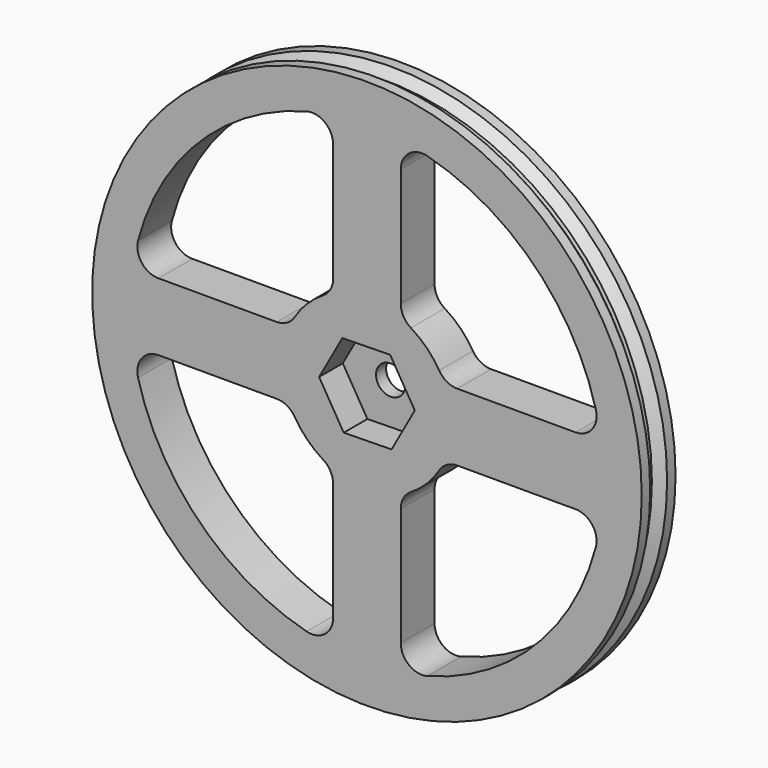
from build123d import *

# Parameters (mm, degrees)
F0_R      = 41.275
F0_R_2    = 40.005
F1_DEPTH  = 3.175
F3_DEPTH  = 4.445
F5_DEPTH  = 6.351
F6_R      = 3.175
F8_D      = 4.4
F9_R      = 41.275
F9_R_2    = 40.005
F10_DEPTH = 1.5875
F11_SIZE  = 1.26999


# Not quite as in the source:
# - a fillet or chamfer is up to 0.001 mm smaller than in the source, because OpenCascade refuses the exact size


with BuildPart() as f1:
    # F0 (on Front) → F1 (new body, symmetric)
    with BuildSketch(Plane.XZ):
        Circle(F0_R)
        Circle(F0_R_2, mode=Mode.SUBTRACT)
        Circle(F0_R_2)
        Polygon((-7.3323484187, 0), (-3.6661742094, 6.35), (3.6661742094, 6.35), (7.3323484187, 0), (3.6661742094, -6.35), (-3.6661742094, -6.35), align=None, mode=Mode.SUBTRACT)
        Polygon((3.6661742094, 6.35), (-3.6661742094, 6.35), (-7.3323484187, 0), (-3.6661742094, -6.35), (3.6661742094, -6.35), (7.3323484187, 0), align=None)
    extrude(amount=F1_DEPTH, both=True)

    # F2 (on face) → F3 (cut)
    with BuildSketch(Plane.XZ.offset(3.175)):
        Polygon((7.1846849266, 0.1208628901), (3.4876721301, 6.2825511097), (-3.6970127965, 6.1616882196), (-7.1846849266, -0.1208628901), (-3.4876721301, -6.2825511097), (3.6970127965, -6.1616882196), align=None)
    extrude(amount=-F3_DEPTH, mode=Mode.SUBTRACT)

    # F4 (on face) → F5 (cut, through all)
    with BuildSketch(Plane.XZ.offset(3.175)):
        with BuildLine():
            ThreePointArc((-35.1952724098, -5.08), (-25.144717139, -25.144717139), (-5.08, -35.1952724098))
            Line((-5.08, -35.1952724098), (-5.08, -11.6397422652))
            ThreePointArc((-5.08, -11.6397422652), (-8.9802561211, -8.9802561211), (-11.6397422652, -5.08))
            Line((-11.6397422652, -5.08), (-35.1952724098, -5.08))
        make_face()
        with BuildLine():
            Line((-5.08, 11.6397422652), (-5.08, 35.1952724098))
            ThreePointArc((-5.08, 35.1952724098), (-25.144717139, 25.144717139), (-35.1952724098, 5.08))
            Line((-35.1952724098, 5.08), (-11.6397422652, 5.08))
            ThreePointArc((-11.6397422652, 5.08), (-8.9802561211, 8.9802561211), (-5.08, 11.6397422652))
        make_face()
        with BuildLine():
            Line((11.6397422652, 5.08), (35.1952724098, 5.08))
            ThreePointArc((35.1952724098, 5.08), (25.144717139, 25.144717139), (5.08, 35.1952724098))
            Line((5.08, 35.1952724098), (5.08, 11.6397422652))
            ThreePointArc((5.08, 11.6397422652), (8.9802561211, 8.9802561211), (11.6397422652, 5.08))
        make_face()
        with BuildLine():
            ThreePointArc((5.08, -35.1952724098), (25.144717139, -25.144717139), (35.1952724098, -5.08))
            Line((35.1952724098, -5.08), (11.6397422652, -5.08))
            ThreePointArc((11.6397422652, -5.08), (8.9802561211, -8.9802561211), (5.08, -11.6397422652))
            Line((5.08, -11.6397422652), (5.08, -35.1952724098))
        make_face()
    extrude(amount=-F5_DEPTH, mode=Mode.SUBTRACT)

    # F6
    f6_edges = [f1.edges().sort_by_distance(p)[0] for p in [
        (-35.195272, 0, -5.08),
        (-11.639742, 0, -5.08),
        (-5.08, 0, -35.195272),
        (-5.08, 0, -11.639742),
        (5.08, 0, -35.195272),
        (5.08, 0, -11.639742),
        (35.195272, 0, -5.08),
        (11.639742, 0, -5.08),
        (-5.08, 0, 35.195272),
        (-5.08, 0, 11.639742),
        (-35.195272, 0, 5.08),
        (-11.639742, 0, 5.08),
        (35.195272, 0, 5.08),
        (11.639742, 0, 5.08),
        (5.08, 0, 35.195272),
        (5.08, 0, 11.639742),
    ]]
    fillet(f6_edges, radius=F6_R)

    # F8 (through all)
    with Locations(Plane.XZ.offset(-1.27)):
        with Locations((0, 0)):
            Hole(F8_D / 2)

    # F9 (on Front) → F10 (cut, symmetric)
    with BuildSketch(Plane.XZ):
        Circle(F9_R)
        Circle(F9_R_2, mode=Mode.SUBTRACT)
    extrude(amount=F10_DEPTH, both=True, mode=Mode.SUBTRACT)

    # F11 (size 1.27 in the source; OpenCascade refuses exactly that, so slightly less here)
    f11_edges = [f1.edges().sort_by_distance(p)[0] for p in [
        (-40.005, 1.5875, 0),
        (-40.005, -1.5875, 0),
    ]]
    chamfer(f11_edges, length=F11_SIZE)


solid = f1.part
